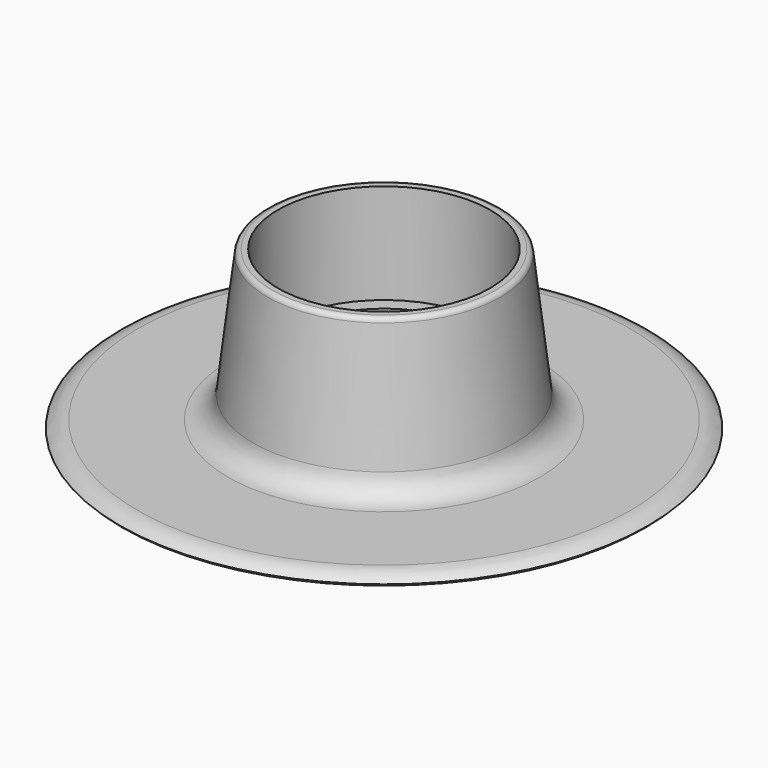
from build123d import *

# Parameters (mm, degrees)
F2_SIZE = 0.5
F4_R    = 1


# Not quite as in the source:
# - a fillet or chamfer that OpenCascade refuses, or shapes differently, is made with other operations: its cross-section is extruded or revolved along the edge and cut away or added


with BuildPart() as f1:
    # F0 (on Front) → F1 (revolve)
    with BuildSketch(Plane.XZ):
        Polygon((23.2, 30), (21.2, 30), (21.2, 10), (18.2991344482, 10), (18.2991344482, 0), (0, 0), (0, -2), (52.7682006359, -2), (52.7682006359, 0), (26.7173200846, 0), align=None)
    revolve(axis=Axis((0, 0, 5.5142873898), (0, 0, -1)))

    # F2
    f2_edges = [f1.edges().sort_by_distance(p)[0] for p in [
        (-52.768201, 0, -2),
    ]]
    chamfer(f2_edges, length=F2_SIZE)

    # F3: fillet of radius 5 on 2 edges, made by hand

    # F3_s1 → F3_t2 (revolve)
    with BuildSketch(Plane.XZ):
        with BuildLine():
            ThreePointArc((31.1653481678, 0), (27.8420335373, 1.2642832191), (26.1993632745, 4.4177680532))
            Line((26.1993632745, 4.4177680532), (26.1000435766, 4.4061234142))
            Line((26.1000435766, 4.4061234142), (26.6283595229, -0.1))
            Line((26.6283595229, -0.1), (31.1653481678, -0.1))
            Line((31.1653481678, -0.1), (31.1653481678, 0))
        make_face()
    revolve(axis=Axis((0, 0, 0), (0, 0, -1)))

    # F3_s3 → F3_t4 (revolve, cut)
    with BuildSketch(Plane.XZ):
        with BuildLine():
            ThreePointArc((52.7682006359, -1.5), (51.1339780947, -0.3902277714), (49.1974864216, 0))
            Line((49.1974864216, 0), (49.1974864216, 0.1))
            Line((49.1974864216, 0.1), (52.7682006359, 0.1))
            Line((52.7682006359, 0.1), (52.8682006359, 0))
            ThreePointArc((52.8682006359, 0), (52.8682006359, -0.75), (52.8396149202, -1.43))
            Line((52.8396149202, -1.43), (52.7682006359, -1.5))
        make_face()
    revolve(axis=Axis((0, 0, 0), (0, 0, -1)), mode=Mode.SUBTRACT)

    # F4
    f4_edges = [f1.edges().sort_by_distance(p)[0] for p in [
        (-23.2, 0, 30),
    ]]
    fillet(f4_edges, radius=F4_R)


solid = f1.part
